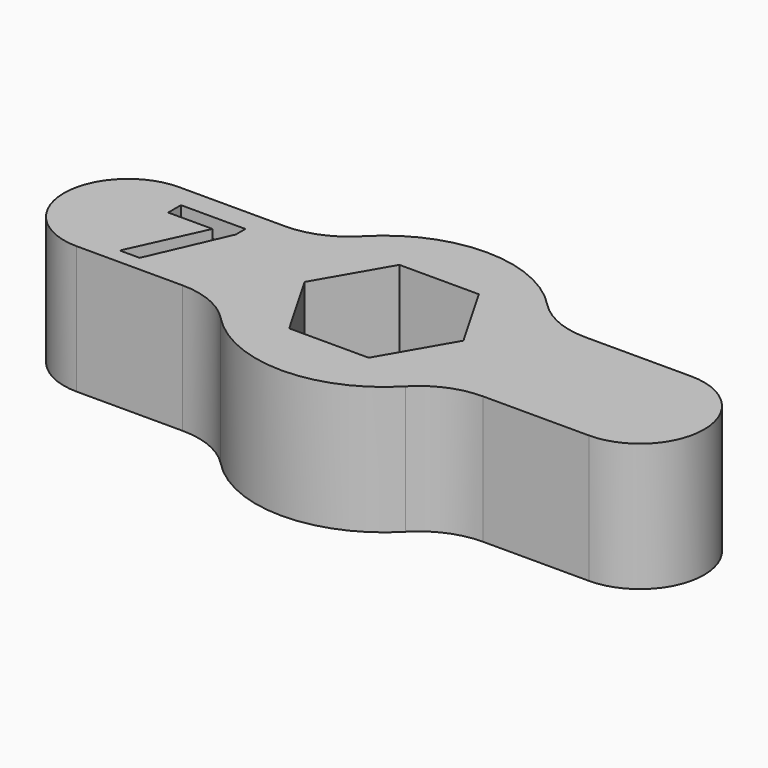
from build123d import *

# Parameters (mm, degrees)
F1_DEPTH     = 8
F2_TEXT_SIZE = 7.8653974924
F3_DEPTH     = 1.2
F4_R         = 5
F5_SIZE      = 0.5


# Not quite as in the source:
# - Text() gives the source's letters only with a copy of the font that has no kerning and outlines rounded to 1/6400 em; it was checked with that copy


with BuildPart() as f1:
    # F0 (on Top) → F1 (new body)
    with BuildSketch(Plane.XY):
        with BuildLine():
            ThreePointArc((-10.9764326567, 0.2955177546), (-12.0482294264, 4.2955177546), (-10.9764326567, 8.2955177546))
            Line((-10.9764326567, 8.2955177546), (-20.0482294264, 8.2955177546))
            ThreePointArc((-20.0482294264, 8.2955177546), (-24.0482294264, 4.2955177546), (-20.0482294264, 0.2955177546))
            Line((-20.0482294264, 0.2955177546), (-10.9764326567, 0.2955177546))
        make_face()
        with BuildLine():
            ThreePointArc((2.8799738039, 0.2955177546), (3.6791771839, 2.2249653937), (3.9517705736, 4.2955177546))
            ThreePointArc((3.9517705736, 4.2955177546), (3.6791771839, 6.3660701154), (2.8799738039, 8.2955177546))
            ThreePointArc((2.8799738039, 8.2955177546), (-4.0482294264, 12.2955177546), (-10.9764326567, 8.2955177546))
            ThreePointArc((-10.9764326567, 8.2955177546), (-12.0482294264, 4.2955177546), (-10.9764326567, 0.2955177546))
            ThreePointArc((-10.9764326567, 0.2955177546), (-4.0482294264, -3.7044822454), (2.8799738039, 0.2955177546))
        make_face()
        Polygon((-1.5656232689, 8.5955177546), (0.9169828886, 4.2955177546), (-1.5656232689, -0.0044822454), (-6.5308355839, -0.0044822454), (-9.0134417414, 4.2955177546), (-6.5308355839, 8.5955177546), align=None, mode=Mode.SUBTRACT)
        with BuildLine():
            ThreePointArc((2.8799738039, 8.2955177546), (3.6791771839, 6.3660701154), (3.9517705736, 4.2955177546))
            ThreePointArc((3.9517705736, 4.2955177546), (3.6791771839, 2.2249653937), (2.8799738039, 0.2955177546))
            Line((2.8799738039, 0.2955177546), (11.9517705736, 0.2955177546))
            ThreePointArc((11.9517705736, 0.2955177546), (15.9517705736, 4.2955177546), (11.9517705736, 8.2955177546))
            Line((11.9517705736, 8.2955177546), (2.8799738039, 8.2955177546))
        make_face()
    extrude(amount=F1_DEPTH)

    # F2 (on face) → F3 (cut)
    with BuildSketch(Plane.XY.offset(8)):
        with Locations((-19.00204923, 1.2564882636)):
            Text('7', F2_TEXT_SIZE, font='Open Sans', font_style=FontStyle.BOLD, text_align=(TextAlign.LEFT, TextAlign.BOTTOM))
    extrude(amount=-F3_DEPTH, mode=Mode.SUBTRACT)

    # F4
    f4_edges = [f1.edges().sort_by_distance(p)[0] for p in [
        (2.879974, 0.295518, 4),
        (-10.976433, 0.295518, 4),
        (2.879974, 8.295518, 4),
        (-10.976433, 8.295518, 4),
    ]]
    fillet(f4_edges, radius=F4_R)

    # F5
    f5_edges = [f1.edges().sort_by_distance(p)[0] for p in [
        (-4.048229, -0.004482, 0),
        (-7.772139, 2.145518, 0),
        (-7.772139, 6.445518, 0),
        (-4.048229, 8.595518, 0),
        (-0.32432, 6.445518, 0),
        (-0.32432, 2.145518, 0),
    ]]
    chamfer(f5_edges, length=F5_SIZE)


solid = f1.part
